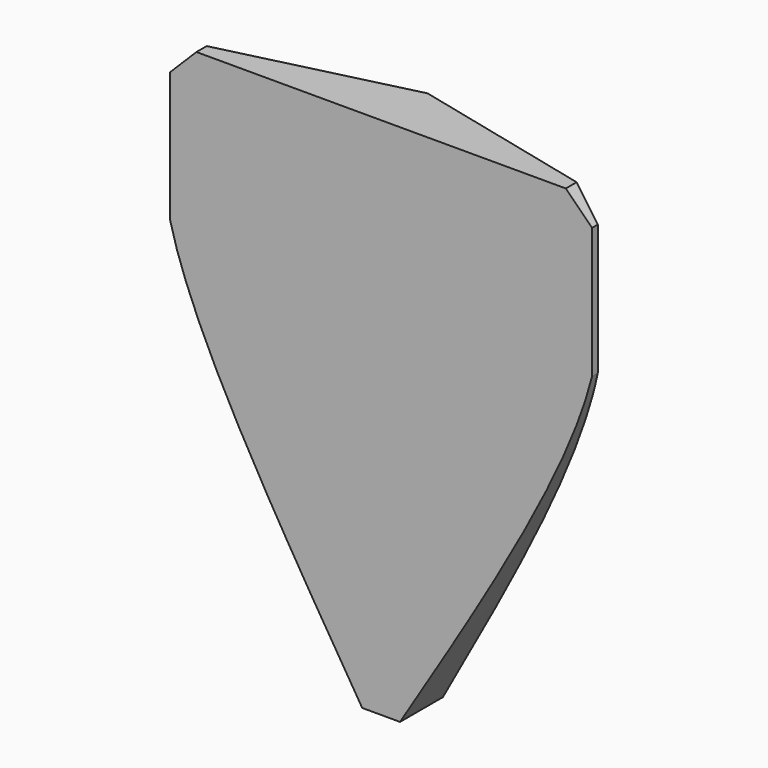
from build123d import *

# Parameters (mm, degrees)
F1_DEPTH = 40
F3_DEPTH = 494


with BuildPart() as f1:
    # F0 (on Front) → F1 (new body)
    with BuildSketch(Plane.XZ):
        with BuildLine():
            add(Edge.make_bspline(
                [(0, 252), (15.8393937026, 187.6250477101), (73.9196968513, 93.8125238551), (132, 0)],
                knots=[0.3599862205, 0.3599862205, 0.3599862205, 0.3599862205, 1, 1, 1, 1], degree=3))
            Line((132, 0), (158, 0))
            add(Edge.make_bspline(
                [(290, 252), (274.1606062974, 187.6250477101), (216.0803031487, 93.8125238551), (158, 0)],
                knots=[0.3599862205, 0.3599862205, 0.3599862205, 0.3599862205, 1, 1, 1, 1], degree=3))
            Line((290, 252), (290, 342))
            Line((290, 342), (272, 360))
            Line((272, 360), (18, 360))
            Line((18, 360), (0, 342))
            Line((0, 342), (0, 252))
        make_face()
    extrude(amount=F1_DEPTH)

    # F2 (on face) → F3 (cut)
    with BuildSketch(Plane.XY.offset(360)):
        Polygon((-17.8489275277, 46.4588217437), (-17.8489275277, -40), (145, 0), (310.4465901852, -40), (307.7366054058, 46.4588217437), align=None)
    extrude(amount=-F3_DEPTH, mode=Mode.SUBTRACT)


solid = f1.part
